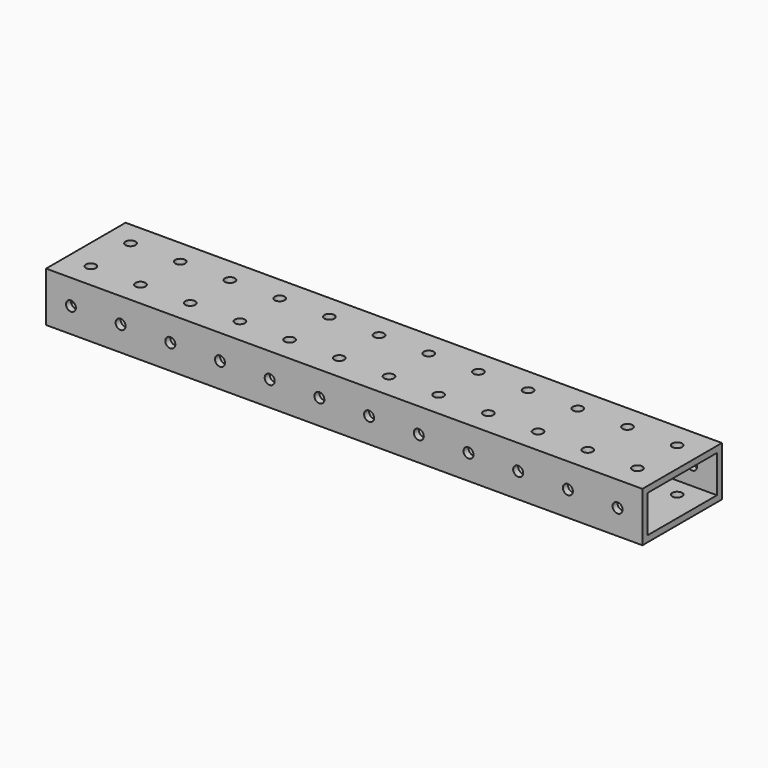
from build123d import *

# Parameters (mm, degrees)
F0_W     = 50.8
F0_H     = 25.4
F0_W_2   = 44.45
F0_H_2   = 19.05
F1_DEPTH = 304.8
F3_D     = 5.1054
F5_D     = 5.1054


# Not quite as in the source:
# - a feature names something its author has since deleted; it is built from what else it names


with BuildPart() as f1:
    # F0 (on Right) → F1 (new body)
    with BuildSketch(Plane.YZ):
        Rectangle(F0_W, F0_H)
        Rectangle(F0_W_2, F0_H_2, mode=Mode.SUBTRACT)
    extrude(amount=F1_DEPTH)

    # F3 (through all)
    with Locations(Plane.XZ.offset(25.4)):
        with Locations((215.9, 0), (63.5, 0), (88.9, 0), (165.1, 0), (38.1, 0), (12.7, 0), (114.3, 0), (292.1, 0), (139.7, 0), (241.3, 0), (190.5, 0), (266.7, 0)):
            Hole(F3_D / 2)

    # F5 (through all)
    with Locations(Plane.XY.offset(12.7)):
        with Locations((114.3, 12.7), (38.1, -12.7), (63.5, 12.7), (38.1, 12.7), (88.9, -12.7), (266.7, -12.7), (215.9, 12.7), (139.7, -12.7), (63.5, -12.7), (190.5, 12.7), (241.3, -12.7), (114.3, -12.7), (12.7, 12.7), (292.1, 12.7), (12.7, -12.7), (190.5, -12.7), (88.9, 12.7), (241.3, 12.7), (165.1, -12.7), (165.1, 12.7), (139.7, 12.7), (266.7, 12.7), (292.1, -12.7), (215.9, -12.7)):
            Hole(F5_D / 2)


solid = f1.part
